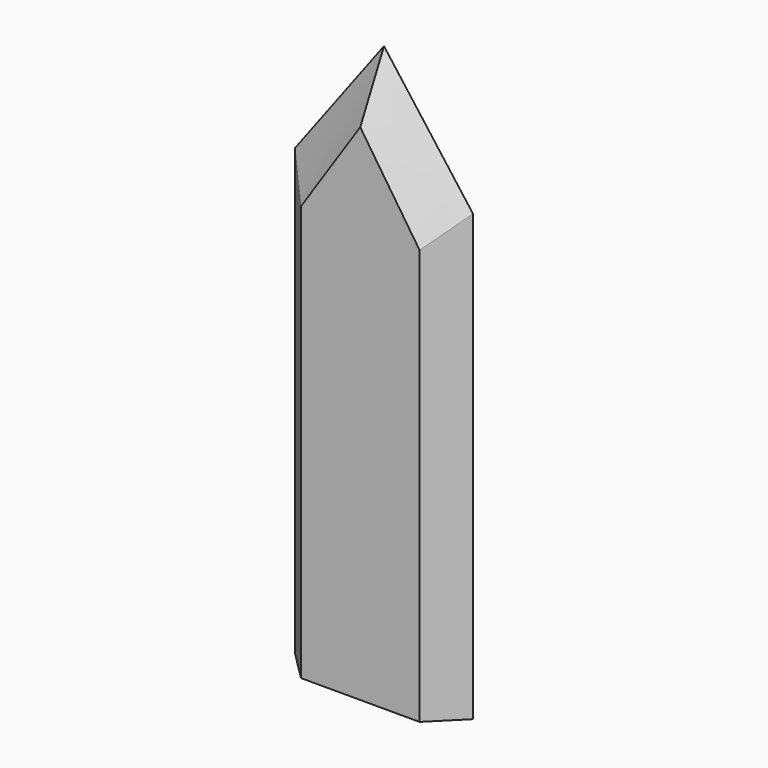
from build123d import *

# Parameters (mm, degrees)
F5_DEPTH = 12.7


with BuildPart() as f3:
    # F0 (on Front) → F3 section 0
    with BuildSketch(Plane.XZ):
        Polygon((-19.05, 0), (0, 0), (19.05, 0), (19.05, 82.55), (0, 107.95), (-19.05, 82.55), align=None)
    # F2 (on offset) → F3 section 1
    with BuildSketch(Plane.XZ.offset(6.35)):
        Polygon((-12.7, 0), (0, 0), (12.7, 0), (12.7, 76.2), (0, 95.25), (-12.7, 76.2), align=None)
    loft()

    # F4 (on face) → F5 (join)
    with BuildSketch(Plane(origin=(0, 0, 0), x_dir=(1, 0, 0), z_dir=(0, 0, -1))):
        with BuildLine():
            Line((-1.0408426169, 0), (0, 0))
            Line((0, 0), (19.05, 0))
            add(Edge.make_bspline(
                [(19.05, 0), (12.7, 6.35)],
                knots=[0, 0, 1, 1], degree=1))
            Line((12.7, 6.35), (-12.7, 6.35))
            add(Edge.make_bspline(
                [(-19.05, 0), (-12.7, 6.35)],
                knots=[0, 0, 1, 1], degree=1))
            Line((-19.05, 0), (-1.0408426169, 0))
        make_face()
    extrude(amount=F5_DEPTH)


solid = f3.part
